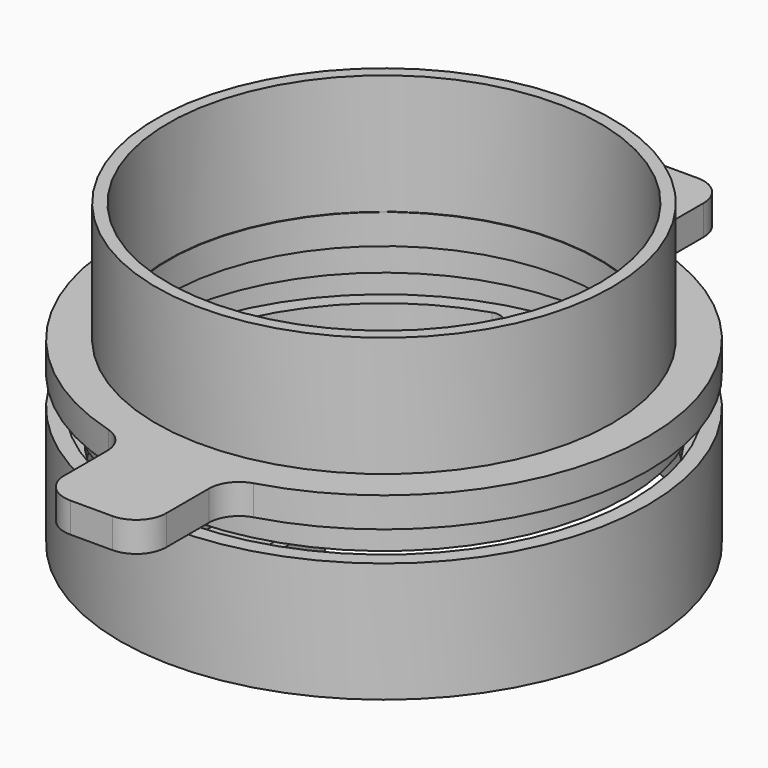
from build123d import *

# Parameters (mm, degrees)
F0_R      = 55.88
F0_R_2    = 52.07
F1_DEPTH  = 12.7
F2_R      = 55.88
F3_DEPTH  = 6.35
F4_R      = 55.88
F4_R_2    = 52.705
F5_DEPTH  = 6.35
F6_W      = 16.51
F6_H      = 16.51
F7_DEPTH  = 4.2333333333
F8_R      = 51.435
F9_DEPTH  = 6.35
F10_R     = 45.56125
F11_DEPTH = 6.35
F12_R     = 48.26
F12_R_2   = 45.72
F13_DEPTH = 25.4
F14_W     = 16.51
F14_H     = 16.51
F15_DEPTH = 4.2333333333


# Not quite as in the source:
# - a length typed as a fraction of an inch, garbled in the dataset ("3 / 203.2 mm" for 3/8 in), is restored


with BuildPart() as f1:
    # F0 (on Top) → F1 (new body)
    with BuildSketch(Plane.XY):
        Circle(F0_R)
        Circle(F0_R_2, mode=Mode.SUBTRACT)
    extrude(amount=F1_DEPTH)

    # F2 (on face) → F3 (join)
    with BuildSketch(Plane.XY.offset(12.7)):
        Circle(F2_R)
        with BuildLine():
            ThreePointArc((-14.9268493151, -47.2272174654), (-49.53, 0), (-14.9268493151, 47.2272174654))
            ThreePointArc((-14.9268493151, 47.2272174654), (-12.09348349, 46.7609468758), (-10.795, 44.1998317304))
            Line((-10.795, 44.1998317304), (-10.795, 30.1625))
            ThreePointArc((-10.795, 30.1625), (-9.8650640303, 27.9174359697), (-7.62, 26.9875))
            Line((-7.62, 26.9875), (7.62, 26.9875))
            ThreePointArc((7.62, 26.9875), (9.8650640303, 27.9174359697), (10.795, 30.1625))
            Line((10.795, 30.1625), (10.795, 44.1998317304))
            ThreePointArc((10.795, 44.1998317304), (12.09348349, 46.7609468758), (14.9268493151, 47.2272174654))
            ThreePointArc((14.9268493151, 47.2272174654), (49.53, 0), (14.9268493151, -47.2272174654))
            ThreePointArc((14.9268493151, -47.2272174654), (12.09348349, -46.7609468758), (10.795, -44.1998317304))
            Line((10.795, -44.1998317304), (10.795, -30.1625))
            ThreePointArc((10.795, -30.1625), (9.8650640303, -27.9174359697), (7.62, -26.9875))
            Line((7.62, -26.9875), (-7.62, -26.9875))
            ThreePointArc((-7.62, -26.9875), (-9.8650640303, -27.9174359697), (-10.795, -30.1625))
            Line((-10.795, -30.1625), (-10.795, -44.1998317304))
            ThreePointArc((-10.795, -44.1998317304), (-12.09348349, -46.7609468758), (-14.9268493151, -47.2272174654))
        make_face(mode=Mode.SUBTRACT)
    extrude(amount=F3_DEPTH)

    # F4 (on face) → F5 (join)
    with BuildSketch(Plane.XY.offset(19.05)):
        Circle(F4_R)
        Circle(F4_R_2, mode=Mode.SUBTRACT)
    extrude(amount=F5_DEPTH)

    # F6 (on face) → F7 (cut)
    with BuildSketch(Plane.XY.offset(19.05)):
        with Locations((0, 38.1)):
            Rectangle(F6_W, F6_H)
        with Locations((0, -38.1)):
            Rectangle(F6_W, F6_H)
    extrude(amount=-F7_DEPTH, mode=Mode.SUBTRACT)


with BuildPart() as f9:
    # F8 (on face) → F9 (new body)
    with BuildSketch(Plane.XY.offset(25.4)):
        Circle(F8_R)
        with BuildLine():
            ThreePointArc((15.905917603, -45.5634654653), (-48.2500123369, -0.9817889236), (14.0392727273, 46.1727887537))
            ThreePointArc((14.0392727273, 46.1727887537), (48.2500123369, 0.9817889236), (15.905917603, -45.5634654653))
        make_face(mode=Mode.SUBTRACT)
    extrude(amount=F9_DEPTH)

    # F10 (on face) → F11 (join)
    with BuildSketch(Plane.XY.offset(31.75)):
        with BuildLine():
            ThreePointArc((-10.795, 59.8215836885), (-12.0739172653, 55.9997228985), (-15.3955102041, 53.717340455))
            ThreePointArc((-15.3955102041, 53.717340455), (-55.88, 0), (-15.3955102041, -53.717340455))
            ThreePointArc((-15.3955102041, -53.717340455), (-12.0739172653, -55.9997228985), (-10.795, -59.8215836885))
            Line((-10.795, -59.8215836885), (-10.795, -71.12))
            ThreePointArc((-10.795, -71.12), (-8.9351280605, -75.6101280605), (-4.445, -77.47))
            Line((-4.445, -77.47), (4.445, -77.47))
            ThreePointArc((4.445, -77.47), (8.9351280605, -75.6101280605), (10.795, -71.12))
            Line((10.795, -71.12), (10.795, -59.8215836885))
            ThreePointArc((10.795, -59.8215836885), (12.0739172653, -55.9997228985), (15.3955102041, -53.717340455))
            ThreePointArc((15.3955102041, -53.717340455), (55.88, 0), (15.3955102041, 53.717340455))
            ThreePointArc((15.3955102041, 53.717340455), (12.0739172653, 55.9997228985), (10.795, 59.8215836885))
            Line((10.795, 59.8215836885), (10.795, 71.12))
            ThreePointArc((10.795, 71.12), (8.9351280605, 75.6101280605), (4.445, 77.47))
            Line((4.445, 77.47), (-4.445, 77.47))
            ThreePointArc((-4.445, 77.47), (-8.9351280605, 75.6101280605), (-10.795, 71.12))
            Line((-10.795, 71.12), (-10.795, 59.8215836885))
        make_face()
        Circle(F10_R, mode=Mode.SUBTRACT)
    extrude(amount=F11_DEPTH)

    # F12 (on face) → F13 (join)
    with BuildSketch(Plane.XY.offset(38.1)):
        Circle(F12_R)
        Circle(F12_R_2, mode=Mode.SUBTRACT)
    extrude(amount=F13_DEPTH)

    # F14 (on face) → F15 (cut)
    with BuildSketch(Plane(origin=(0, 0, 31.75), x_dir=(1, 0, 0), z_dir=(0, 0, -1))):
        with Locations((0, -62.23)):
            Rectangle(F14_W, F14_H)
        with Locations((0, 62.23)):
            Rectangle(F14_W, F14_H)
    extrude(amount=-F15_DEPTH, mode=Mode.SUBTRACT)


solid = Compound([f1.part, f9.part])
